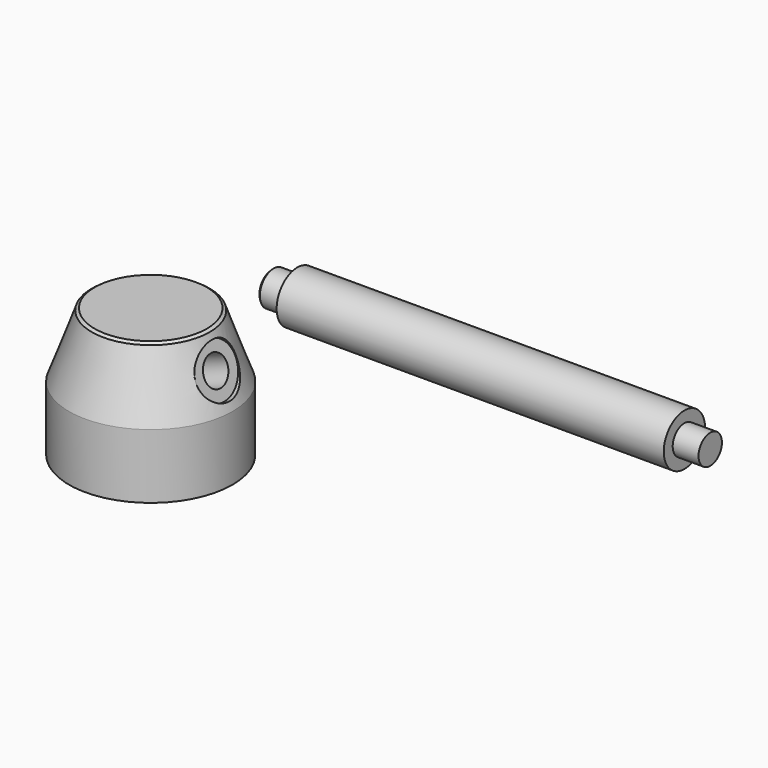
from build123d import *

# Parameters (mm, degrees)
F0_R       = 19
F1_DEPTH   = 15
F1_TAPER   = 20
F2_DEPTH   = 15
F6_R       = 6
F7_DEPTH   = 1.25
F8_D       = 6.8
F8_DEPTH   = 10
F8_TIP     = 2.0429261047
F10_D      = 18.5
F10_DEPTH  = 15
F10_TIP    = 5.557960726
F11_R      = 4
F12_DEPTH  = 6
F11_R_2    = 6
F12_FACE_R = 4
F13_DEPTH  = 90
F14_SIZE   = 0.5
F15_R      = 3.4
F16_DEPTH  = 6


# Not quite as in the source:
# - a fillet or chamfer that OpenCascade refuses, or shapes differently, is made with other operations: its cross-section is extruded or revolved along the edge and cut away or added
# - the program builds the solid bodies; features that only make, move or delete a surface that nothing else refers to are left out


with BuildPart() as f1:
    # F0 (on Top) → F1 (new body)
    with BuildSketch(Plane.XY):
        Circle(F0_R)
    extrude(amount=F1_DEPTH, taper=F1_TAPER)

    # F2 (add): a face of the model
    f2_faces = [f1.faces().sort_by_distance(p)[0] for p in [
        (0, 0, 0),
    ]]
    extrude(f2_faces, amount=F2_DEPTH)

    # F4: chamfer of 0.5 on 1 edges, made by hand

    # F4_s1 → F4_t2 (revolve, cut)
    with BuildSketch(Plane.XZ):
        Polygon((13.7114565577, 14.5301536896), (13.040446486, 15), (13.540446486, 15), align=None)
    revolve(axis=Axis((0, 0, 15), (0, 0, -1)), mode=Mode.SUBTRACT)

    # F6 (on line) → F7 (cut)
    with BuildSketch(Plane(origin=(16.7774222096, 0, 6.106482292), x_dir=(0, -1, 0), z_dir=(-0.9396926208, 0, -0.3420201433))):
        with Locations((0, 1.4829505704)):
            Circle(F6_R)
    extrude(amount=F7_DEPTH, mode=Mode.SUBTRACT)

    # F8
    with Locations(Plane(origin=(16.7774222096, 0, 6.106482292), x_dir=(0, -1, 0), z_dir=(0.9396926208, 0, 0.3420201433))):
        with Locations((0, -1.4829505704)):
            Hole(F8_D / 2, depth=F8_DEPTH)
            with Locations((0, 0, -(F8_DEPTH + F8_TIP / 2))):  # 118° drill point
                Cone(0, F8_D / 2, F8_TIP, mode=Mode.SUBTRACT)

    # F10
    with Locations(Plane(origin=(0, 0, -15), x_dir=(1, 0, 0), z_dir=(0, 0, -1))):
        with Locations((0, 0)):
            Hole(F10_D / 2, depth=F10_DEPTH)
            with Locations((0, 0, -(F10_DEPTH + F10_TIP / 2))):  # 118° drill point
                Cone(0, F10_D / 2, F10_TIP, mode=Mode.SUBTRACT)


with BuildPart() as f12:
    # F11 (on Right) → F12 (new body)
    with BuildSketch(Plane.YZ):
        with Locations((42.5821989775, 0)):
            Circle(F11_R)
    extrude(amount=-F12_DEPTH)

    # F11 (on Right) + F12_face (on face) → F13 (join)
    with BuildSketch(Plane.YZ):
        with Locations((42.5821989775, 0)):
            Circle(F11_R_2)
        with Locations((42.5821989775, 0)):
            Circle(F11_R, mode=Mode.SUBTRACT)
    with BuildSketch(Plane(origin=(0, 42.5821989775, 0), x_dir=(0, 1, 0), z_dir=(1, 0, 0))):
        Circle(F12_FACE_R)
    extrude(amount=F13_DEPTH)

    # F14
    f14_edges = [f12.edges().sort_by_distance(p)[0] for p in [
        (-6, 38.582199, 0),
    ]]
    chamfer(f14_edges, length=F14_SIZE)

    # F15 (on face) → F16 (join)
    with BuildSketch(Plane.YZ.offset(90)):
        with Locations((42.5821989775, 0)):
            Circle(F15_R)
    extrude(amount=F16_DEPTH)


solid = Compound([f1.part, f12.part])
